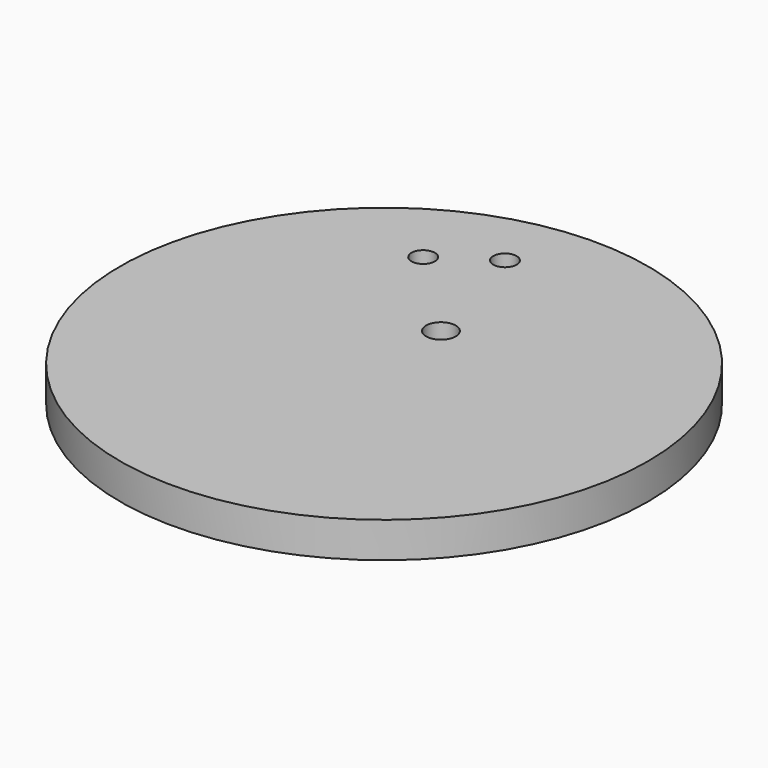
from build123d import *

# Parameters (mm, degrees)
F0_R     = 148.5
F0_R_2   = 6.5786
F0_R_3   = 8.3312
F1_DEPTH = 20
F2_R     = 146.5
F2_R_2   = 142
F3_DEPTH = 5


# Not quite as in the source:
# - a feature names something its author has since deleted; it is built from what else it names


with BuildPart() as f1:
    # F0 (on Top) → F1 (new body)
    with BuildSketch(Plane.XY):
        Circle(F0_R)
        with Locations((-50, 90)):
            Circle(F0_R_2, mode=Mode.SUBTRACT)
        with Locations((-20, 110)):
            Circle(F0_R_2, mode=Mode.SUBTRACT)
        with Locations((0, 40)):
            Circle(F0_R_3, mode=Mode.SUBTRACT)
    extrude(amount=F1_DEPTH)

    # F2 (on face) → F3 (cut)
    with BuildSketch(Plane.XY):
        Circle(F2_R)
        Circle(F2_R_2, mode=Mode.SUBTRACT)
    extrude(amount=F3_DEPTH, mode=Mode.SUBTRACT)


solid = f1.part
